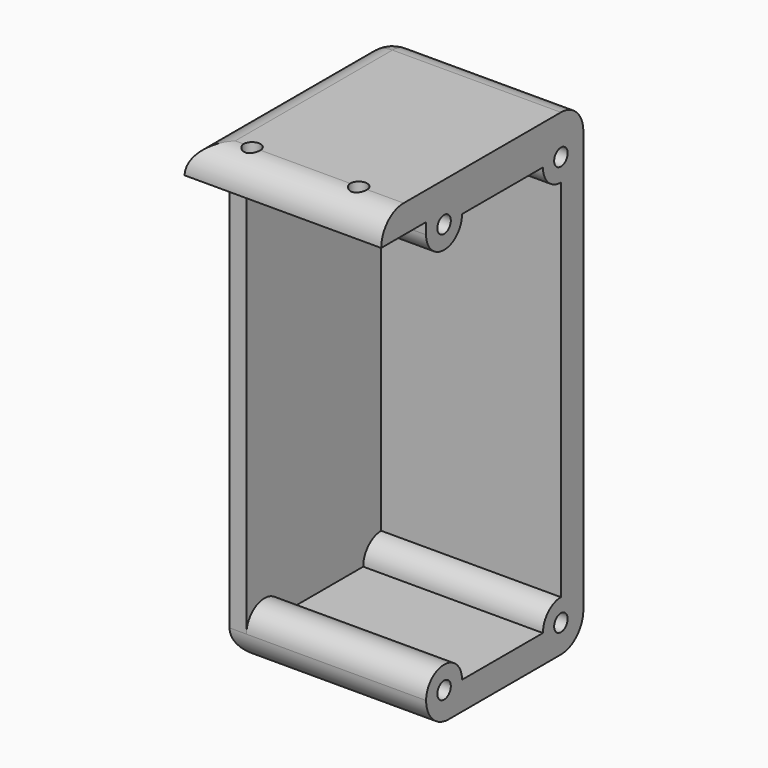
from build123d import *

# Parameters (mm, degrees)
F1_DEPTH     = 17.5
F3_DEPTH     = 3
F5_D         = 3
F5_DEPTH     = 25
F5_TIP       = 0.9012909285
F7_D         = 3
F7_DEPTH     = 25
F7_TIP       = 0.9012909285
F8_T1_DEPTH  = 60
F8_T3_DEPTH  = 42.5
F8_T5_DEPTH  = 75
F8_T7_DEPTH  = 42.5
F8_T9_DEPTH  = 52.5
F8_S13_W     = 5
F8_S13_H     = 5
F8_T14_DEPTH = 5
F8_S19_W     = 5
F8_S19_H     = 5
F8_T20_DEPTH = 5


# Not quite as in the source:
# - a fillet or chamfer that OpenCascade refuses, or shapes differently, is made with other operations: its cross-section is extruded or revolved along the edge and cut away or added


with BuildPart() as f1:
    # F0 (on Right) → F1 (new body, symmetric)
    with BuildSketch(Plane.YZ):
        Polygon((-2.2390836586, 4.4176964641), (-2.2390836586, -0.5823035359), (7.7609163414, -0.5823035359), (7.7609163414, -2.5823035359), (15.7609163414, -2.5823035359), (33.7609163414, -2.5823035359), (37.7609163414, -2.5823035359), (37.7609163414, -6.5823035359), (37.7609163414, -71.5823035359), (37.7609163414, -75.5823035359), (33.7609163414, -75.5823035359), (15.7609163414, -75.5823035359), (7.7609163414, -75.5823035359), (7.7609163414, -80.5823035359), (42.7609163414, -80.5823035359), (42.7609163414, 4.4176964641), align=None)
        with BuildLine():
            Line((15.7609163414, -2.5823035359), (7.7609163414, -2.5823035359))
            ThreePointArc((7.7609163414, -2.5823035359), (11.7609163414, -6.5823035359), (15.7609163414, -2.5823035359))
        make_face()
        with BuildLine():
            Line((37.7609163414, -2.5823035359), (33.7609163414, -2.5823035359))
            ThreePointArc((33.7609163414, -2.5823035359), (34.9324892166, -5.4107306607), (37.7609163414, -6.5823035359))
            Line((37.7609163414, -6.5823035359), (37.7609163414, -2.5823035359))
        make_face()
        with BuildLine():
            ThreePointArc((15.7609163414, -75.5823035359), (11.7609163414, -71.5823035359), (7.7609163414, -75.5823035359))
            Line((7.7609163414, -75.5823035359), (15.7609163414, -75.5823035359))
        make_face()
        with BuildLine():
            Line((37.7609163414, -75.5823035359), (37.7609163414, -71.5823035359))
            ThreePointArc((37.7609163414, -71.5823035359), (34.9324892166, -72.7538764112), (33.7609163414, -75.5823035359))
            Line((33.7609163414, -75.5823035359), (37.7609163414, -75.5823035359))
        make_face()
    extrude(amount=F1_DEPTH, both=True)

    # F2 (on face) → F3 (join)
    with BuildSketch(Plane(origin=(-17.5, 0, 0), x_dir=(0, -1, 0), z_dir=(-1, 0, 0))):
        with BuildLine():
            Line((-7.7609163414, -75.5823035359), (-7.7609163414, -2.5823035359))
            ThreePointArc((-7.7609163414, -2.5823035359), (-11.7609163414, -6.5823035359), (-15.7609163414, -2.5823035359))
            Line((-15.7609163414, -2.5823035359), (-33.7609163414, -2.5823035359))
            ThreePointArc((-33.7609163414, -2.5823035359), (-34.9324892166, -5.4107306607), (-37.7609163414, -6.5823035359))
            Line((-37.7609163414, -6.5823035359), (-37.7609163414, -71.5823035359))
            ThreePointArc((-37.7609163414, -71.5823035359), (-34.9324892166, -72.7538764112), (-33.7609163414, -75.5823035359))
            Line((-33.7609163414, -75.5823035359), (-15.7609163414, -75.5823035359))
            ThreePointArc((-15.7609163414, -75.5823035359), (-11.7609163414, -71.5823035359), (-7.7609163414, -75.5823035359))
        make_face()
    extrude(amount=-F3_DEPTH)

    # F5
    with Locations(Plane.YZ.offset(17.5)):
        with Locations((11.7609163414, -2.5823035359), (37.7609163414, -2.5823035359), (37.7609163414, -75.5823035359), (11.7609163414, -75.5823035359)):
            Hole(F5_D / 2, depth=F5_DEPTH)
            with Locations((0, 0, -(F5_DEPTH + F5_TIP / 2))):  # 118° drill point
                Cone(0, F5_D / 2, F5_TIP, mode=Mode.SUBTRACT)

    # F7
    with Locations(Plane.XY.offset(4.4176964641)):
        with Locations((-9.5, 2.7609163414), (9.5, 2.7609163414)):
            Hole(F7_D / 2, depth=F7_DEPTH)
            with Locations((0, 0, -(F7_DEPTH + F7_TIP / 2))):  # 118° drill point
                Cone(0, F7_D / 2, F7_TIP, mode=Mode.SUBTRACT)

    # F8: fillet of radius 5 on 7 edges, made by hand

    # F8_s2 → F8_t1 (cut)
    with BuildSketch(Plane.YZ.offset(-30)):
        with BuildLine():
            ThreePointArc((2.7609163414, 4.4176964641), (-0.7746175645, 2.95323037), (-2.2390836586, -0.5823035359))
            Line((-2.2390836586, -0.5823035359), (-2.2390836586, 4.4176964641))
            Line((-2.2390836586, 4.4176964641), (2.7609163414, 4.4176964641))
        make_face()
        with BuildLine():
            ThreePointArc((7.7609163414, -75.5823035359), (9.2253824355, -79.1178374419), (12.7609163414, -80.5823035359))
            Line((12.7609163414, -80.5823035359), (7.7609163414, -80.5823035359))
            Line((7.7609163414, -80.5823035359), (7.7609163414, -75.5823035359))
        make_face()
    extrude(amount=F8_T1_DEPTH, mode=Mode.SUBTRACT)

    # F8_s4 → F8_t3 (cut)
    with BuildSketch(Plane.YZ.offset(-12.5)):
        with BuildLine():
            ThreePointArc((42.7609163414, -0.5823035359), (41.2964502473, 2.95323037), (37.7609163414, 4.4176964641))
            Line((37.7609163414, 4.4176964641), (42.7609163414, 4.4176964641))
            Line((42.7609163414, 4.4176964641), (42.7609163414, -0.5823035359))
        make_face()
        with BuildLine():
            ThreePointArc((37.7609163414, -80.5823035359), (41.2964502473, -79.1178374419), (42.7609163414, -75.5823035359))
            Line((42.7609163414, -75.5823035359), (42.7609163414, -80.5823035359))
            Line((42.7609163414, -80.5823035359), (37.7609163414, -80.5823035359))
        make_face()
    extrude(amount=F8_T3_DEPTH, mode=Mode.SUBTRACT)

    # F8_s6 → F8_t5 (cut)
    with BuildSketch(Plane.XY.offset(-75.5823035359)):
        with BuildLine():
            ThreePointArc((-17.5, 37.7609163414), (-16.0355339059, 41.2964502473), (-12.5, 42.7609163414))
            Line((-12.5, 42.7609163414), (-17.5, 42.7609163414))
            Line((-17.5, 42.7609163414), (-17.5, 37.7609163414))
        make_face()
    extrude(amount=F8_T5_DEPTH, mode=Mode.SUBTRACT)

    # F8_s8 → F8_t7 (cut)
    with BuildSketch(Plane.XZ.offset(-37.7609163414)):
        with BuildLine():
            ThreePointArc((-12.5, -80.5823035359), (-16.0355339059, -79.1178374419), (-17.5, -75.5823035359))
            Line((-17.5, -75.5823035359), (-17.5, -80.5823035359))
            Line((-17.5, -80.5823035359), (-12.5, -80.5823035359))
        make_face()
    extrude(amount=F8_T7_DEPTH, mode=Mode.SUBTRACT)

    # F8_s10 → F8_t9 (cut)
    with BuildSketch(Plane.XZ.offset(-37.7609163414)):
        with BuildLine():
            ThreePointArc((-17.5, -0.5823035359), (-16.0355339059, 2.95323037), (-12.5, 4.4176964641))
            Line((-12.5, 4.4176964641), (-17.5, 4.4176964641))
            Line((-17.5, 4.4176964641), (-17.5, -0.5823035359))
        make_face()
    extrude(amount=F8_T9_DEPTH, mode=Mode.SUBTRACT)


with BuildPart() as f8_tool12:
    # F8_s13 → F8_t14 (new body)
    with BuildSketch(Plane.XZ.offset(-37.7609163414)):
        with Locations((-15, 1.9176964641)):
            Rectangle(F8_S13_W, F8_S13_H)
    extrude(amount=-F8_T14_DEPTH)

    # F8_s15 → F8_t16 (revolve, cut)
    with BuildSketch(Plane(origin=(-12.5, 37.7609163414, -0.5823035359), x_dir=(0.7071067812, 0, -0.7071067812), z_dir=(0.7071067812, 0, 0.7071067812))):
        with BuildLine():
            ThreePointArc((0, -5), (5, 0), (0, 5))
            Line((0, 5), (0, -5))
        make_face()
    revolve(axis=Axis((-12.5, 37.7609163414, -0.5823035359), (0, 1, 0)), mode=Mode.SUBTRACT)


with BuildPart() as f1_1:
    add(f1.part)

    # F8_t11: cut F8_tool12
    add(f8_tool12.part, mode=Mode.SUBTRACT)


with BuildPart() as f8_tool18:
    # F8_s19 → F8_t20 (new body)
    with BuildSketch(Plane.XZ.offset(-37.7609163414)):
        with Locations((-15, -78.0823035359)):
            Rectangle(F8_S19_W, F8_S19_H)
    extrude(amount=-F8_T20_DEPTH)

    # F8_s21 → F8_t22 (revolve, cut)
    with BuildSketch(Plane(origin=(-12.5, 37.7609163414, -75.5823035359), x_dir=(0.7071067812, 0, 0.7071067812), z_dir=(-0.7071067812, 0, 0.7071067812))):
        with BuildLine():
            ThreePointArc((0, -5), (5, 0), (0, 5))
            Line((0, 5), (0, -5))
        make_face()
    revolve(axis=Axis((-12.5, 37.7609163414, -75.5823035359), (0, 1, 0)), mode=Mode.SUBTRACT)


with BuildPart() as f1_2:
    add(f1_1.part)

    # F8_t17: cut F8_tool18
    add(f8_tool18.part, mode=Mode.SUBTRACT)


solid = f1_2.part
